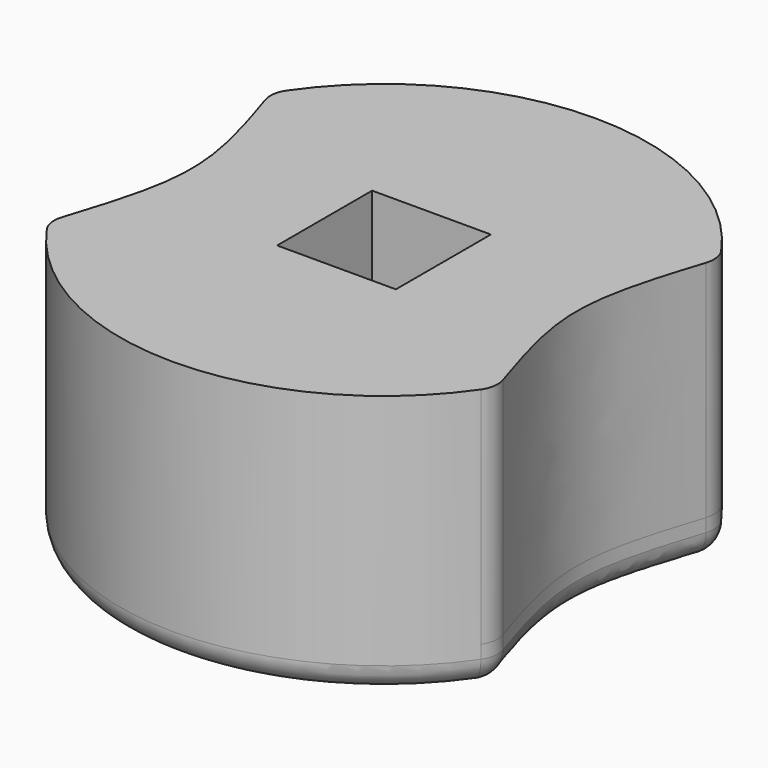
from build123d import *
from build123d import SkipClean  # not in build123d's __all__

# Parameters (mm, degrees)
F0_W     = 9
F0_H     = 9
F1_DEPTH = 3
F2_DEPTH = 20
F3_DEPTH = 25
F4_R     = 2


with BuildPart() as f1:
    # F0 (on Top) → F1 (new body)
    with BuildSketch(Plane.XY):
        with BuildLine():
            ThreePointArc((17, -10.5356537529), (19.2353840617, -5.4772255751), (20, 0))
            ThreePointArc((20, 0), (19.2353840617, 5.4772255751), (17, 10.5356537529))
            add(Edge.make_bspline(
                [(17, -10.5356537529), (15.4390588775, -5.7747014672), (13.767943494, 0), (15.4390588775, 5.7747014672), (17, 10.5356537529)],
                knots=[0, 0, 0, 0, 0.5, 1, 1, 1, 1], degree=3))
        make_face()
        with BuildLine():
            add(Edge.make_bspline(
                [(17, -10.5356537529), (15.4390588775, -5.7747014672), (13.767943494, 0), (15.4390588775, 5.7747014672), (17, 10.5356537529)],
                knots=[0, 0, 0, 0, 0.5, 1, 1, 1, 1], degree=3))
            ThreePointArc((17, 10.5356537529), (0, 20), (-17, 10.5356537529))
            add(Edge.make_bspline(
                [(-17, -10.5356537529), (-15.4390588775, -5.7747014672), (-13.767943494, 0), (-15.4390588775, 5.7747014672), (-17, 10.5356537529)],
                knots=[0, 0, 0, 0, 0.5, 1, 1, 1, 1], degree=3))
            ThreePointArc((-17, -10.5356537529), (0, -20), (17, -10.5356537529))
        make_face()
        Rectangle(F0_W, F0_H, mode=Mode.SUBTRACT)
        with BuildLine():
            add(Edge.make_bspline(
                [(-17, -10.5356537529), (-15.4390588775, -5.7747014672), (-13.767943494, 0), (-15.4390588775, 5.7747014672), (-17, 10.5356537529)],
                knots=[0, 0, 0, 0, 0.5, 1, 1, 1, 1], degree=3))
            ThreePointArc((-17, 10.5356537529), (-20, 0), (-17, -10.5356537529))
        make_face()
        Rectangle(F0_W, F0_H)
    extrude(amount=F1_DEPTH)

    # F0 (on Top) → F2 (join)
    with BuildSketch(Plane.XY):
        with BuildLine():
            add(Edge.make_bspline(
                [(17, -10.5356537529), (15.4390588775, -5.7747014672), (13.767943494, 0), (15.4390588775, 5.7747014672), (17, 10.5356537529)],
                knots=[0, 0, 0, 0, 0.5, 1, 1, 1, 1], degree=3))
            ThreePointArc((17, 10.5356537529), (0, 20), (-17, 10.5356537529))
            add(Edge.make_bspline(
                [(-17, -10.5356537529), (-15.4390588775, -5.7747014672), (-13.767943494, 0), (-15.4390588775, 5.7747014672), (-17, 10.5356537529)],
                knots=[0, 0, 0, 0, 0.5, 1, 1, 1, 1], degree=3))
            ThreePointArc((-17, -10.5356537529), (0, -20), (17, -10.5356537529))
        make_face()
        Rectangle(F0_W, F0_H, mode=Mode.SUBTRACT)
    with SkipClean():  # cleaning this boolean's faces spoils the solid; the shape is the same uncleaned
        extrude(amount=F2_DEPTH)

    # F0 (on Top) → F3 (cut)
    with BuildSketch(Plane.XY):
        with BuildLine():
            add(Edge.make_bspline(
                [(-17, -10.5356537529), (-15.4390588775, -5.7747014672), (-13.767943494, 0), (-15.4390588775, 5.7747014672), (-17, 10.5356537529)],
                knots=[0, 0, 0, 0, 0.5, 1, 1, 1, 1], degree=3))
            ThreePointArc((-17, 10.5356537529), (-20, 0), (-17, -10.5356537529))
        make_face()
        with BuildLine():
            ThreePointArc((17, -10.5356537529), (19.2353840617, -5.4772255751), (20, 0))
            ThreePointArc((20, 0), (19.2353840617, 5.4772255751), (17, 10.5356537529))
            add(Edge.make_bspline(
                [(17, -10.5356537529), (15.4390588775, -5.7747014672), (13.767943494, 0), (15.4390588775, 5.7747014672), (17, 10.5356537529)],
                knots=[0, 0, 0, 0, 0.5, 1, 1, 1, 1], degree=3))
        make_face()
    extrude(amount=F3_DEPTH, mode=Mode.SUBTRACT)

    # F4
    f4_edges = [f1.edges().sort_by_distance(p)[0] for p in [
        (0, 20, 0),
        (-14.603501, 0, 0),
        (0, -20, 0),
        (14.603501, 0, 0),
        (-17, 10.535654, 1.5),
        (-17, 10.535654, 11.5),
        (-17, -10.535654, 1.5),
        (-17, -10.535654, 11.5),
        (17, 10.535654, 1.5),
        (17, 10.535654, 11.5),
        (17, -10.535654, 11.5),
        (17, -10.535654, 1.5),
    ]]
    fillet(f4_edges, radius=F4_R)


solid = f1.part
